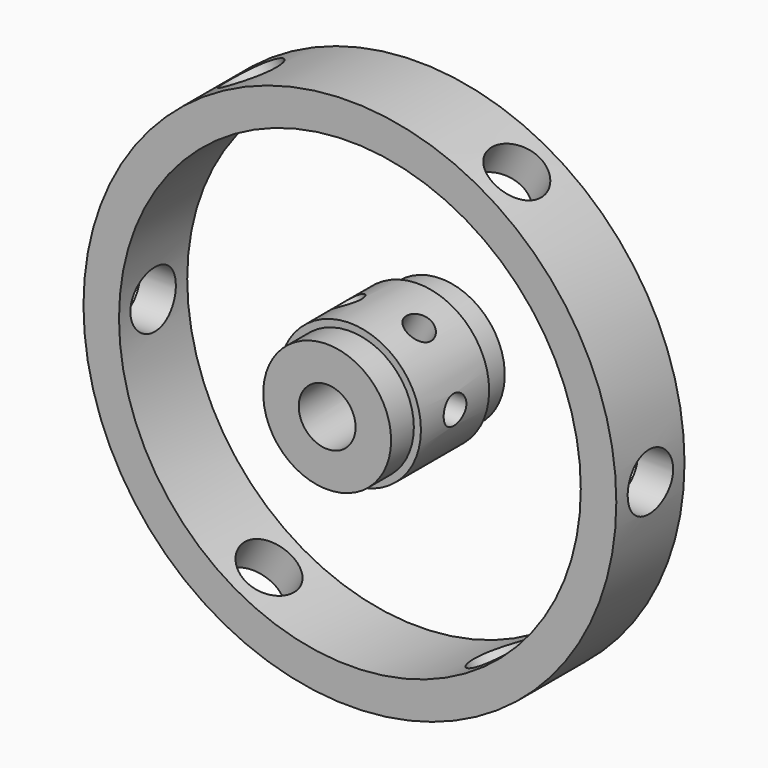
from build123d import *

# Parameters (mm, degrees)
F0_R      = 37.5
F0_R_2    = 32.5
F1_DEPTH  = 6
F3_R      = 4
F4_DEPTH  = 115
F7_R      = 4
F8_DEPTH  = 40
F10_R     = 4
F11_DEPTH = 40
F12_R     = 10
F12_R_2   = 4
F13_DEPTH = 10
F14_R     = 12.415089
F14_R_2   = 9
F15_DEPTH = 4
F16_R     = 12.379451
F16_R_2   = 9
F17_DEPTH = 4
F18_R     = 2
F19_DEPTH = 12.5
F20_R     = 2
F21_DEPTH = 25
F22_R     = 2
F23_DEPTH = 25


with BuildPart() as f1:
    # F0 (on Front) → F1 (new body, symmetric)
    with BuildSketch(Plane.XZ):
        Circle(F0_R)
        Circle(F0_R_2, mode=Mode.SUBTRACT)
    extrude(amount=F1_DEPTH, both=True)

    # F3 (on offset) → F4 (cut)
    with BuildSketch(Plane.YZ.offset(37.5)):
        Circle(F3_R)
    extrude(amount=-F4_DEPTH, mode=Mode.SUBTRACT)

    # F7 (on face) → F8 (cut, symmetric)
    with BuildSketch(Plane(origin=(0, 0, 0), x_dir=(0.866025, 0, 0.5), z_dir=(0.5, 0, -0.866025))):
        Circle(F7_R)
    extrude(amount=F8_DEPTH, both=True, mode=Mode.SUBTRACT)

    # F10 (on face) → F11 (cut, symmetric)
    with BuildSketch(Plane(origin=(0, 0, 0), x_dir=(0.866025, 0, -0.5), z_dir=(-0.5, 0, -0.866025))):
        Circle(F10_R)
    extrude(amount=F11_DEPTH, both=True, mode=Mode.SUBTRACT)


with BuildPart() as f13:
    # F12 (on Front) → F13 (new body, symmetric)
    with BuildSketch(Plane.XZ):
        Circle(F12_R)
        Circle(F12_R_2, mode=Mode.SUBTRACT)
    extrude(amount=F13_DEPTH, both=True)

    # F14 (on face) → F15 (cut)
    with BuildSketch(Plane.XZ.offset(10)):
        Circle(F14_R)
        Circle(F14_R_2, mode=Mode.SUBTRACT)
    extrude(amount=-F15_DEPTH, mode=Mode.SUBTRACT)

    # F16 (on face) → F17 (cut)
    with BuildSketch(Plane(origin=(0, 10, 0), x_dir=(-1, 0, 0), z_dir=(0, 1, 0))):
        Circle(F16_R)
        Circle(F16_R_2, mode=Mode.SUBTRACT)
    extrude(amount=-F17_DEPTH, mode=Mode.SUBTRACT)

    # F18 (on Right) → F19 (cut, symmetric)
    with BuildSketch(Plane.YZ):
        Circle(F18_R)
    extrude(amount=F19_DEPTH, both=True, mode=Mode.SUBTRACT)

    # F20 (on face) → F21 (cut)
    with BuildSketch(Plane(origin=(0, 0, 0), x_dir=(0.866025, 0, 0.5), z_dir=(0.5, 0, -0.866025))):
        Circle(F20_R)
    extrude(amount=-F21_DEPTH, mode=Mode.SUBTRACT)

    # F22 (on face) → F23 (cut)
    with BuildSketch(Plane(origin=(0, 0, 0), x_dir=(0.866025, 0, -0.5), z_dir=(-0.5, 0, -0.866025))):
        Circle(F22_R)
    extrude(amount=-F23_DEPTH, mode=Mode.SUBTRACT)


solid = Compound([f1.part, f13.part])
